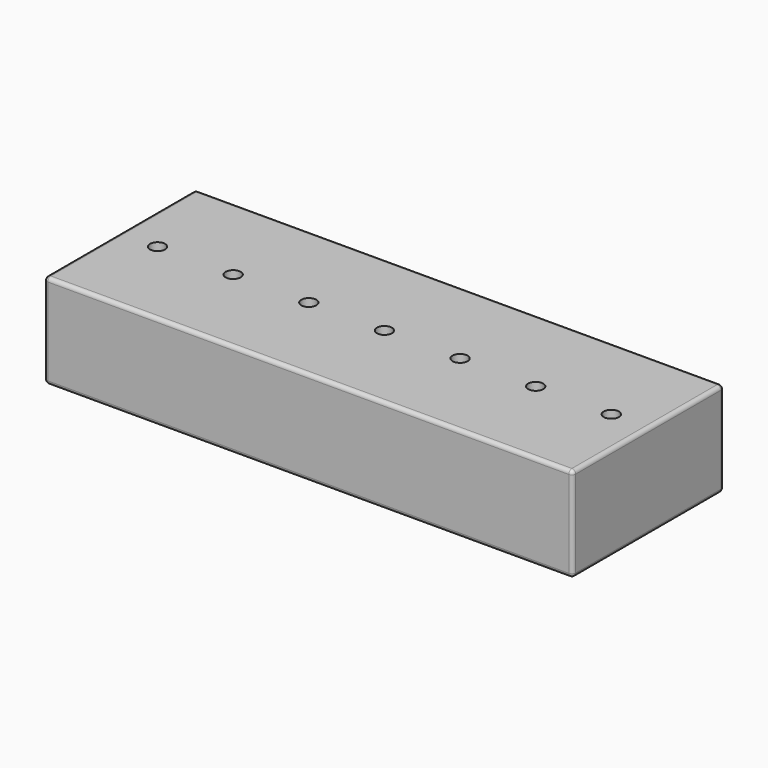
from build123d import *

# Parameters (mm, degrees)
F0_W     = 71.0019436256
F0_H     = 25.4
F0_R     = 1.016
F1_DEPTH = 12.7
F2_R     = 0.508


# Not quite as in the source:
# - a feature names something its author has since deleted; it is built from what else it names


with BuildPart() as f1:
    # F0 (on Top) → F1 (new body)
    with BuildSketch(Plane.XY):
        with Locations((-26.4490794038, 5.7338142046)):
            Rectangle(F0_W, F0_H)
        with Locations((-56.8700512166, 5.7338142046)):
            Circle(F0_R, mode=Mode.SUBTRACT)
        with Locations((-46.7100512166, 5.7338142046)):
            Circle(F0_R, mode=Mode.SUBTRACT)
        with Locations((-36.5500512166, 5.7338142046)):
            Circle(F0_R, mode=Mode.SUBTRACT)
        with Locations((-26.3900512166, 5.7338142046)):
            Circle(F0_R, mode=Mode.SUBTRACT)
        with Locations((-16.2300512166, 5.7338142046)):
            Circle(F0_R, mode=Mode.SUBTRACT)
        with Locations((-6.0700512166, 5.7338142046)):
            Circle(F0_R, mode=Mode.SUBTRACT)
        with Locations((4.0899487834, 5.7338142046)):
            Circle(F0_R, mode=Mode.SUBTRACT)
    extrude(amount=-F1_DEPTH)

    # F2
    f2_edges = [f1.edges().sort_by_distance(p)[0] for p in [
        (-26.449079, 18.433814, 0),
        (-26.449079, -6.966186, 0),
        (-61.950051, 5.733814, 0),
        (-61.950051, -6.966186, -6.35),
        (-61.950051, 18.433814, -6.35),
        (-26.449079, 18.433814, -12.7),
        (-61.950051, 5.733814, -12.7),
        (-26.449079, -6.966186, -12.7),
        (9.051892, 5.733814, -12.7),
        (9.051892, 5.733814, 0),
        (9.051892, 18.433814, -6.35),
        (9.051892, -6.966186, -6.35),
    ]]
    fillet(f2_edges, radius=F2_R)


solid = f1.part
